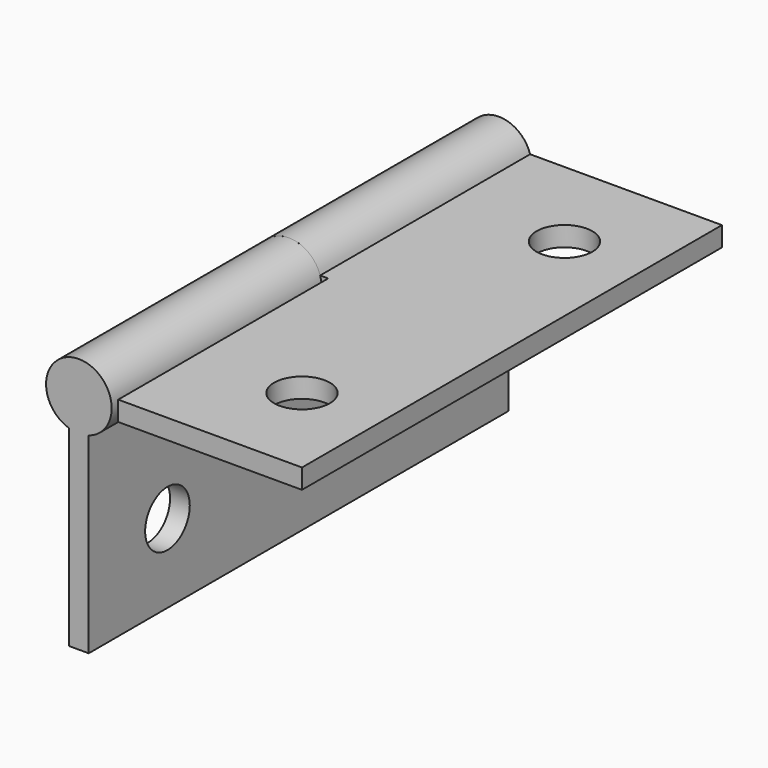
from build123d import *

# Parameters (mm, degrees)
F0_R      = 5
F1_DEPTH  = 40
F2_R      = 3
F3_DEPTH  = 40
F5_W      = 3
F5_H      = 80
F6_DEPTH  = 30
F7_R      = 5
F7_R_2    = 3
F8_DEPTH  = 40
F10_W     = 80
F10_H     = 3
F11_DEPTH = 30
F12_W     = 40
F12_H     = 2
F13_DEPTH = 25
F14_W     = 2
F14_H     = 40
F15_DEPTH = 25
F16_R     = 4.25
F17_DEPTH = 25
F18_R     = 4.25
F19_DEPTH = 25


with BuildPart() as f1:
    # F0 (on Front) → F1 (new body)
    with BuildSketch(Plane.XZ):
        Circle(F0_R)
    extrude(amount=F1_DEPTH)

    # F2 (on Front) → F3 (join)
    with BuildSketch(Plane.XZ):
        Circle(F2_R)
    extrude(amount=-F3_DEPTH)

    # F5 (on offset) → F6 (join)
    with BuildSketch(Plane.XY.offset(-4)):
        Rectangle(F5_W, F5_H)
    extrude(amount=-F6_DEPTH)

    # F12 (on face) → F13 (cut)
    with BuildSketch(Plane.YZ.offset(1.5)):
        with Locations((20, -5)):
            Rectangle(F12_W, F12_H)
    extrude(amount=-F13_DEPTH, mode=Mode.SUBTRACT)

    # F18 (on face) → F19 (cut)
    with BuildSketch(Plane.YZ.offset(1.5)):
        with Locations((-25, -22)):
            Circle(F18_R)
        with Locations((25, -22)):
            Circle(F18_R)
    extrude(amount=-F19_DEPTH, mode=Mode.SUBTRACT)


with BuildPart() as f8:
    # F7 (on Front) → F8 (new body)
    with BuildSketch(Plane.XZ):
        Circle(F7_R)
        Circle(F7_R_2, mode=Mode.SUBTRACT)
    extrude(amount=-F8_DEPTH)

    # F10 (on offset) → F11 (join)
    with BuildSketch(Plane.YZ.offset(4)):
        Rectangle(F10_W, F10_H)
    extrude(amount=F11_DEPTH)

    # F14 (on face) → F15 (cut)
    with BuildSketch(Plane(origin=(0, 0, -1.5), x_dir=(1, 0, 0), z_dir=(0, 0, -1))):
        with Locations((5, 20)):
            Rectangle(F14_W, F14_H)
    extrude(amount=-F15_DEPTH, mode=Mode.SUBTRACT)

    # F16 (on face) → F17 (cut)
    with BuildSketch(Plane(origin=(0, 0, -1.5), x_dir=(1, 0, 0), z_dir=(0, 0, -1))):
        with Locations((22, 25)):
            Circle(F16_R)
        with Locations((22, -25)):
            Circle(F16_R)
    extrude(amount=-F17_DEPTH, mode=Mode.SUBTRACT)


solid = Compound([f1.part, f8.part])
